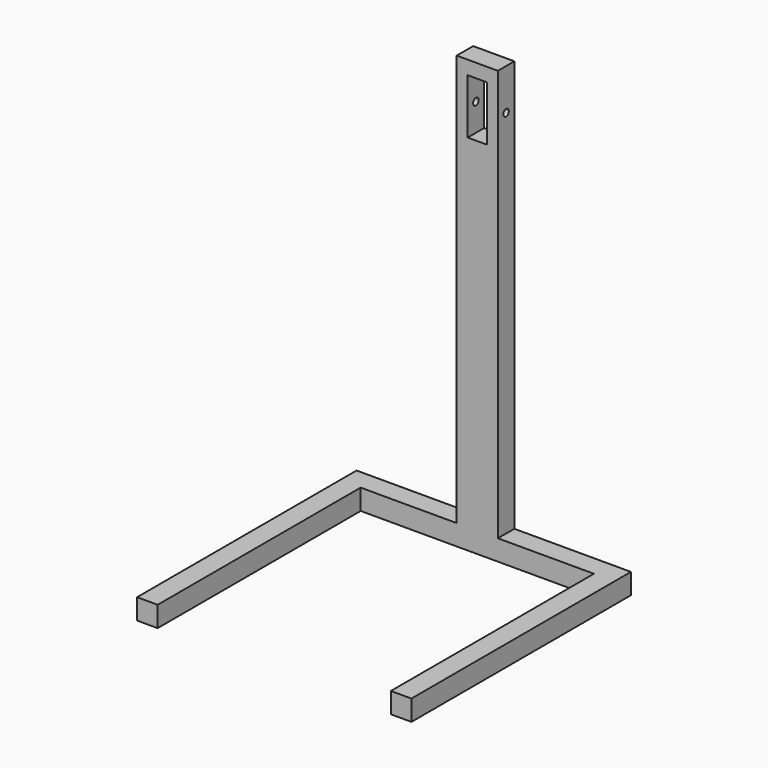
from build123d import *

# Parameters (mm, degrees)
F1_DEPTH  = 75
F2_W      = 150
F2_H      = 75
F3_DEPTH  = 1500
F4_W      = 70
F4_H      = 200
F5_DEPTH  = 75.001
F6_W      = 6
F6_H      = 20
F7_DEPTH  = 40
F8_R      = 9.99999
F9_R      = 3.25
F10_DEPTH = 507.501
F12_R     = 12.5
F13_DEPTH = 575.001


# Not quite as in the source:
# - a fillet or chamfer is up to 0.001 mm smaller than in the source, because OpenCascade refuses the exact size
# - a feature of the source that left no trace in its solid (it failed there, or was rolled back) is left out


with BuildPart() as f1:
    # F0 (on Top) → F1 (new body)
    with BuildSketch(Plane.XY):
        Polygon((500, 0), (-500, 0), (-500, -1000), (-425, -1000), (-425, -75), (425, -75), (425, -1000), (500, -1000), align=None)
    extrude(amount=F1_DEPTH)

    # F2 (on face) → F3 (join)
    with BuildSketch(Plane.XY.offset(75)):
        with Locations((0, -37.5)):
            Rectangle(F2_W, F2_H)
    extrude(amount=F3_DEPTH)

    # F4 (on face) → F5 (cut, through all)
    with BuildSketch(Plane.XZ.offset(75)):
        with Locations((0, 1425)):
            Rectangle(F4_W, F4_H)
    extrude(amount=-F5_DEPTH, mode=Mode.SUBTRACT)

    # F6 (on face) → F7 (join)
    with BuildSketch(Plane(origin=(0, 0, 0), x_dir=(-1, 0, 0), z_dir=(0, 1, 0))):
        with Locations((-4.5, 710)):
            Rectangle(F6_W, F6_H)
        with Locations((10.5, 710)):
            Rectangle(F6_W, F6_H)
    extrude(amount=F7_DEPTH)

    # F8 (radius 10 in the source; OpenCascade refuses exactly that, so slightly less here)
    f8_edges = [f1.edges().sort_by_distance(p)[0] for p in [
        (4.5, 40, 720),
        (4.5, 40, 700),
        (-10.5, 40, 720),
        (-10.5, 40, 700),
    ]]
    fillet(f8_edges, radius=F8_R)

    # F9 (on face) → F10 (cut, through all)
    with BuildSketch(Plane.YZ.offset(7.5)):
        with Locations((31, 710)):
            Circle(F9_R)
    extrude(amount=-F10_DEPTH, mode=Mode.SUBTRACT)

    # F12 (on face) → F13 (cut, through all)
    with BuildSketch(Plane(origin=(-75, 0, 0), x_dir=(0, -1, 0), z_dir=(-1, 0, 0))):
        with Locations((37.5, 1425)):
            Circle(F12_R)
    extrude(amount=-F13_DEPTH, mode=Mode.SUBTRACT)


solid = f1.part
